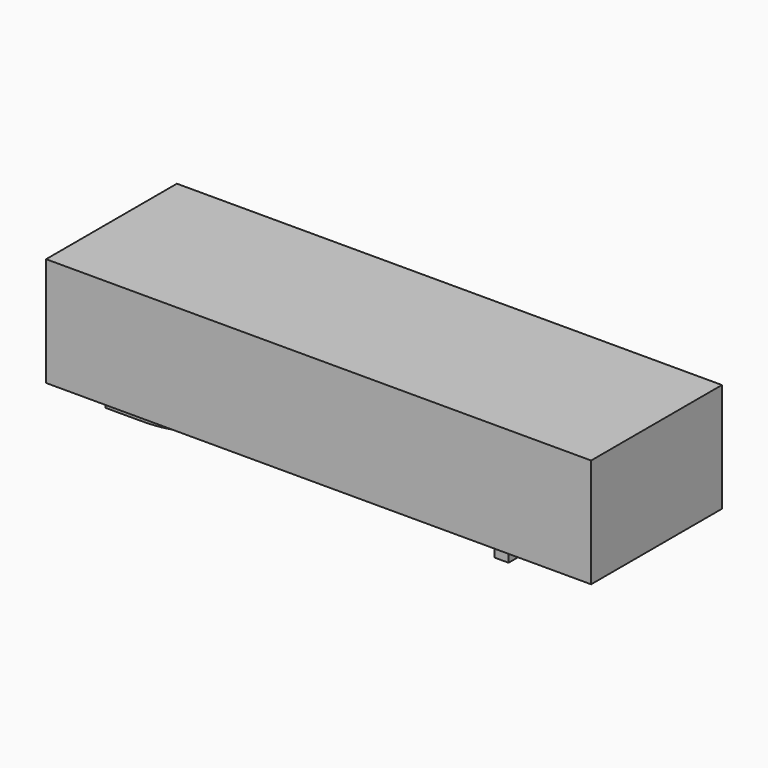
from build123d import *

# Parameters (mm, degrees)
F0_W         = 500
F0_H         = 100
F1_DEPTH     = 150
F2_TEXT_SIZE = 158.647647024
F3_DEPTH     = 15


# Not quite as in the source:
# - Text() gives the source's letters only with a copy of the font that has no kerning and outlines rounded to 1/6400 em; it was checked with that copy


with BuildPart() as f1:
    # F0 (on Front) → F1 (new body)
    with BuildSketch(Plane.XZ):
        with Locations((40.845866483, 11.3943675533)):
            Rectangle(F0_W, F0_H)
    extrude(amount=F1_DEPTH)

    # F2 (on face) → F3 (join)
    with BuildSketch(Plane(origin=(0, 0, -38.6056324467), x_dir=(1, 0, 0), z_dir=(0, 0, -1))):
        with Locations((-185.4601353407, 17.7701320499)):
            Text('Bench', F2_TEXT_SIZE, font='Open Sans', text_align=(TextAlign.LEFT, TextAlign.BOTTOM))
    extrude(amount=F3_DEPTH)


solid = f1.part
